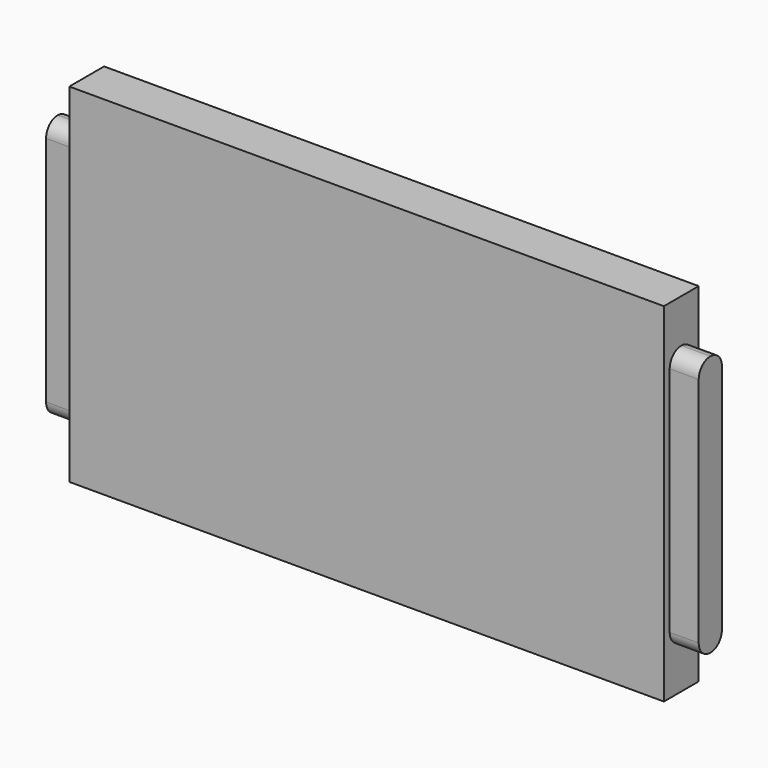
from build123d import *

# Parameters (mm, degrees)
F0_W     = 260.35
F0_H     = 19.05
F1_DEPTH = 152.4
F2_W     = 12.7
F2_H     = 114.3
F3_DEPTH = 12.7
F4_R     = 6.34999
F5_W     = 12.7
F5_H     = 114.3
F6_DEPTH = 12.7
F7_R     = 6.34999


# Not quite as in the source:
# - a fillet or chamfer is up to 0.001 mm smaller than in the source, because OpenCascade refuses the exact size


with BuildPart() as f1:
    # F0 (on Top) → F1 (new body)
    with BuildSketch(Plane.XY):
        Rectangle(F0_W, F0_H)
    extrude(amount=-F1_DEPTH)

    # F2 (on face) → F3 (join)
    with BuildSketch(Plane(origin=(-130.175, 0, 0), x_dir=(0, -1, 0), z_dir=(-1, 0, 0))):
        with Locations((0, -76.2)):
            Rectangle(F2_W, F2_H)
    extrude(amount=F3_DEPTH)

    # F4 (radius 6.35 in the source; OpenCascade refuses exactly that, so slightly less here)
    f4_edges = [f1.edges().sort_by_distance(p)[0] for p in [
        (-136.525, 6.35, -19.05),
        (-136.525, -6.35, -19.05),
        (-136.525, -6.35, -133.35),
        (-136.525, 6.35, -133.35),
    ]]
    fillet(f4_edges, radius=F4_R)

    # F5 (on face) → F6 (join)
    with BuildSketch(Plane.YZ.offset(130.175)):
        with Locations((0, -76.2)):
            Rectangle(F5_W, F5_H)
    extrude(amount=F6_DEPTH)

    # F7 (radius 6.35 in the source; OpenCascade refuses exactly that, so slightly less here)
    f7_edges = [f1.edges().sort_by_distance(p)[0] for p in [
        (136.525, -6.35, -19.05),
        (136.525, 6.35, -19.05),
        (136.525, 6.35, -133.35),
        (136.525, -6.35, -133.35),
    ]]
    fillet(f7_edges, radius=F7_R)


solid = f1.part
